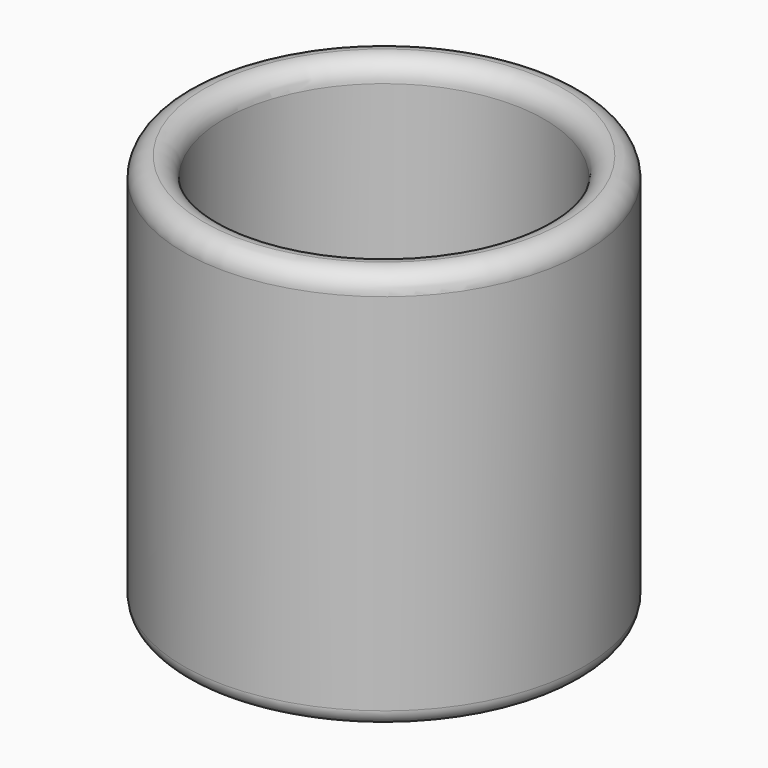
from build123d import *

# Parameters (mm, degrees)
F2_R = 6.34999
F3_R = 5.08


# Not quite as in the source:
# - a fillet or chamfer is up to 0.001 mm smaller than in the source, because OpenCascade refuses the exact size


with BuildPart() as f1:
    # F0 (on Front) → F1 (revolve)
    with BuildSketch(Plane.XZ):
        Polygon((-63.5, 0), (0, 0), (0, 12.7), (-50.8, 12.7), (-50.8, 127), (-63.5, 127), align=None)
    revolve(axis=Axis((0, 0, 6.35), (0, 0, -1)))

    # F2 (radius 6.35 in the source; OpenCascade refuses exactly that, so slightly less here)
    f2_edges = [f1.edges().sort_by_distance(p)[0] for p in [
        (63.5, 0, 127),
        (50.8, 0, 127),
    ]]
    fillet(f2_edges, radius=F2_R)

    # F3
    f3_edges = [f1.edges().sort_by_distance(p)[0] for p in [
        (63.5, 0, 0),
    ]]
    fillet(f3_edges, radius=F3_R)


solid = f1.part
